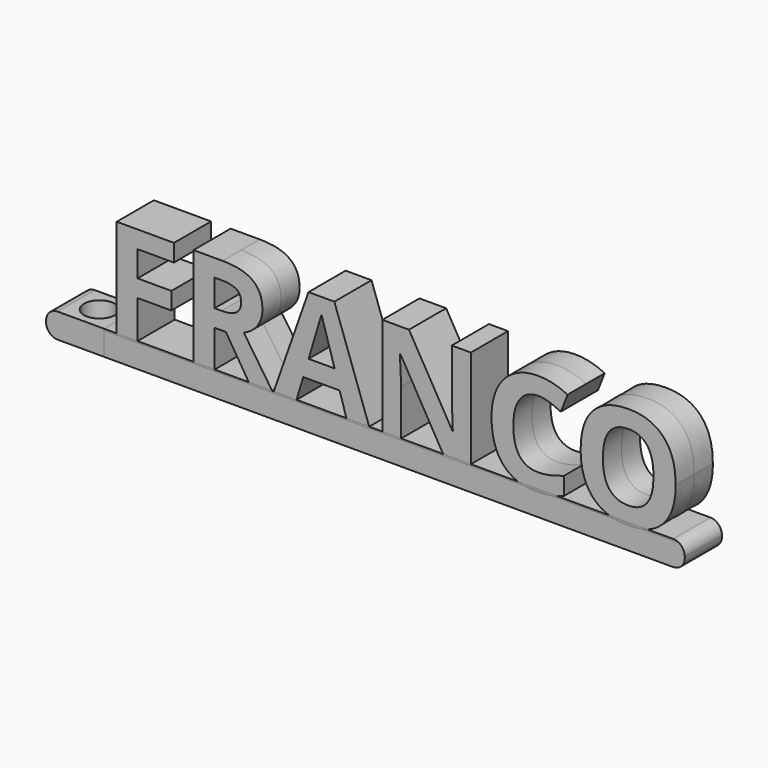
from build123d import *

# Parameters (mm, degrees)
F0_TEXT_SIZE = 18.0641276532
F1_DEPTH     = 3
F2_W         = 75
F2_H         = 6
F3_DEPTH     = 0.2
F4_DEPTH     = 3
F5_W         = 6
F5_H         = 3.2
F6_DEPTH     = 7.5
F7_R         = 1.5
F8_R         = 2
F9_DEPTH     = 3.5
F10_T1_DEPTH = 13.5


# Not quite as in the source:
# - a fillet or chamfer that OpenCascade refuses, or shapes differently, is made with other operations: its cross-section is extruded or revolved along the edge and cut away or added
# - Text() gives the source's letters only with a copy of the font that has no kerning and outlines rounded to 1/6400 em; it was checked with that copy


with BuildPart() as f1:
    # F0 (on Front) → F1 (new body, symmetric)
    with BuildSketch(Plane.XZ):
        with Locations((-20, 0)):
            Text('FRANCO', F0_TEXT_SIZE, font='Open Sans', font_style=FontStyle.BOLD, text_align=(TextAlign.LEFT, TextAlign.BOTTOM))
    extrude(amount=F1_DEPTH, both=True)



with BuildPart() as f3:
    # F2 (on Top) → F3 (new body)
    with BuildSketch(Plane.XY):
        with Locations((17.5, 0)):
            Rectangle(F2_W, F2_H)
    extrude(amount=F3_DEPTH)


with BuildPart() as f4:
    # F4 (new): a face of the model
    f4_faces = [f3.part.faces().sort_by_distance(p)[0] for p in [
        (17.5, 0, 0),
    ]]
    extrude(f4_faces, amount=F4_DEPTH)


with BuildPart() as f1_1:
    add(f1.part)

    add(f3.part)  # F6 merges F3

    add(f4.part)  # F6 merges F4
    # F5 (on face) → F6 (join)
    with BuildSketch(Plane(origin=(-20, 0, 0), x_dir=(0, -1, 0), z_dir=(-1, 0, 0))):
        with Locations((0, -1.4)):
            Rectangle(F5_W, F5_H)
    extrude(amount=F6_DEPTH)

    # F7
    f7_edges = [f1_1.edges().sort_by_distance(p)[0] for p in [
        (-27.5, 0, -3),
        (-27.5, 0, 0.2),
        (55, 0, -3),
    ]]
    fillet(f7_edges, radius=F7_R)

    # F8 (on face) → F9 (cut)
    with BuildSketch(Plane.XY.offset(0.2)):
        with Locations((-23, 0)):
            Circle(F8_R)
    extrude(amount=-F9_DEPTH, mode=Mode.SUBTRACT)

    # F10: fillet of radius 1.5 on 1 edges, made by hand

    # F10_s2 → F10_t1 (cut)
    with BuildSketch(Plane.XZ.offset(-6.75)):
        with BuildLine():
            ThreePointArc((55, -1.3), (54.5606601718, -0.2393398282), (53.5, 0.2))
            Line((53.5, 0.2), (55, 0.2))
            Line((55, 0.2), (55, -1.3))
        make_face()
    extrude(amount=F10_T1_DEPTH, mode=Mode.SUBTRACT)


solid = f1_1.part
